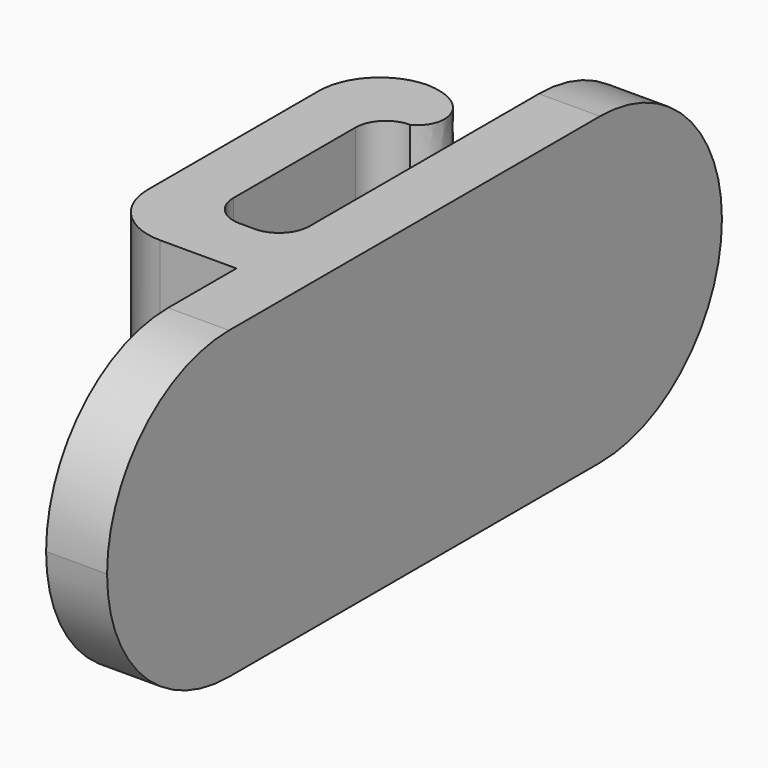
from build123d import *

# Parameters (mm, degrees)
F1_DEPTH      = 10
F2_W          = 2
F2_H          = 10
F3_DEPTH      = 13.3
F3_DEPTH_BACK = 11.9
F4_R          = 4.99999


# Not quite as in the source:
# - a fillet or chamfer is up to 0.001 mm smaller than in the source, because OpenCascade refuses the exact size


with BuildPart() as f1:
    # F0 (on Top) → F1 (new body)
    with BuildSketch(Plane.XY):
        with BuildLine():
            Line((-1.25, -5.5), (3.25, -5.5))
            Line((3.25, -5.5), (3.25, 3.499999999))
            ThreePointArc((3.25, 3.499999999), (2.2500000005, 4.499999999), (1.25, 3.5))
            Line((1.25, 3.5), (1.25, -2.5))
            ThreePointArc((1.25, -2.5), (0.9571067812, -3.2071067812), (0.25, -3.5))
            Line((0.25, -3.5), (-0.25, -3.5))
            ThreePointArc((-0.25, -3.5), (-0.9571067812, -3.2071067812), (-1.25, -2.5))
            Line((-1.25, -2.5), (-1.25, 2.5))
            ThreePointArc((-1.25, 2.5), (-0.9571067812, 3.2071067812), (-0.25, 3.5))
            add(Edge.make_bspline(
                [(-1.2744928417, 5.5), (0.3231141309, 5.4264482222), (0.6423479063, 3.9560622536), (-0.25, 3.5)],
                knots=[0, 0, 0, 0, 2.2471282969, 2.2471282969, 2.2471282969, 2.2471282969], degree=3))
            ThreePointArc((-1.2744928417, 5.5), (-2.6728467387, 4.9056773399), (-3.25, 3.5001499804))
            Line((-3.25, 3.5001499804), (-3.25, -3.5))
            ThreePointArc((-3.25, -3.5), (-2.6642135624, -4.9142135624), (-1.25, -5.5))
        make_face()
    extrude(amount=F1_DEPTH)

    # F2 (on Front) → F3 (join, two sides)
    with BuildSketch(Plane.XZ) as f3_sk:
        with Locations((2.25, 5)):
            Rectangle(F2_W, F2_H)
    extrude(amount=F3_DEPTH)
    extrude(f3_sk.sketch, amount=-F3_DEPTH_BACK)

    # F4 (radius 5 in the source; OpenCascade refuses exactly that, so slightly less here)
    f4_edges = [f1.edges().sort_by_distance(p)[0] for p in [
        (2.25, -13.3, 10),
        (2.25, 11.9, 10),
        (2.25, -13.3, 0),
        (2.25, 11.9, 0),
    ]]
    fillet(f4_edges, radius=F4_R)


solid = f1.part
